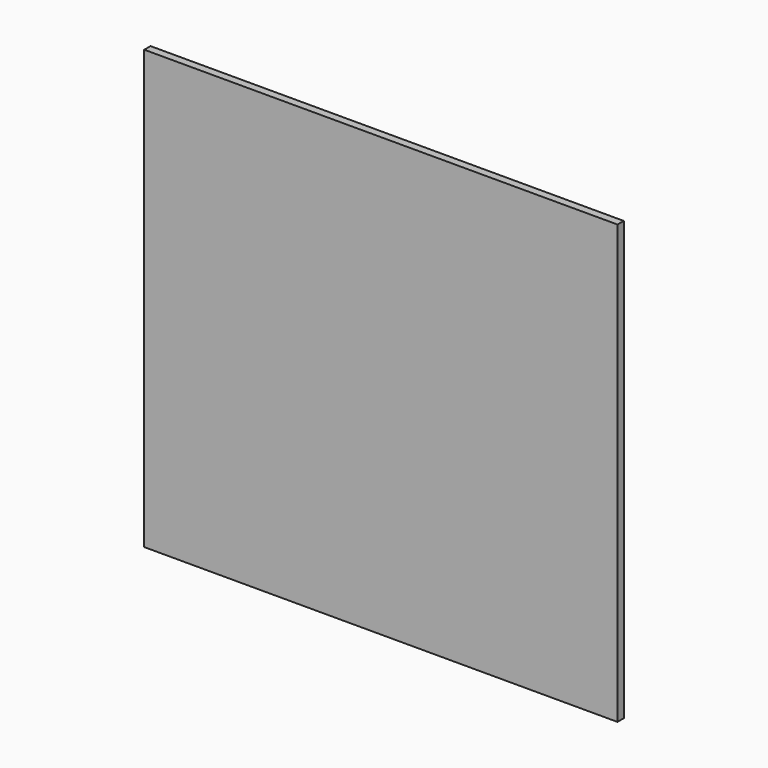
from build123d import *

# Parameters (mm, degrees)
F0_W     = 241
F0_H     = 223
F1_DEPTH = 4


# Not quite as in the source:
# - a feature names something its author has since deleted; it is built from what else it names


with BuildPart() as f1:
    # F0 (on Front) → F1 (new body)
    with BuildSketch(Plane.XZ):
        with Locations((120.5, 111.5)):
            Rectangle(F0_W, F0_H)
    extrude(amount=F1_DEPTH)


solid = f1.part
